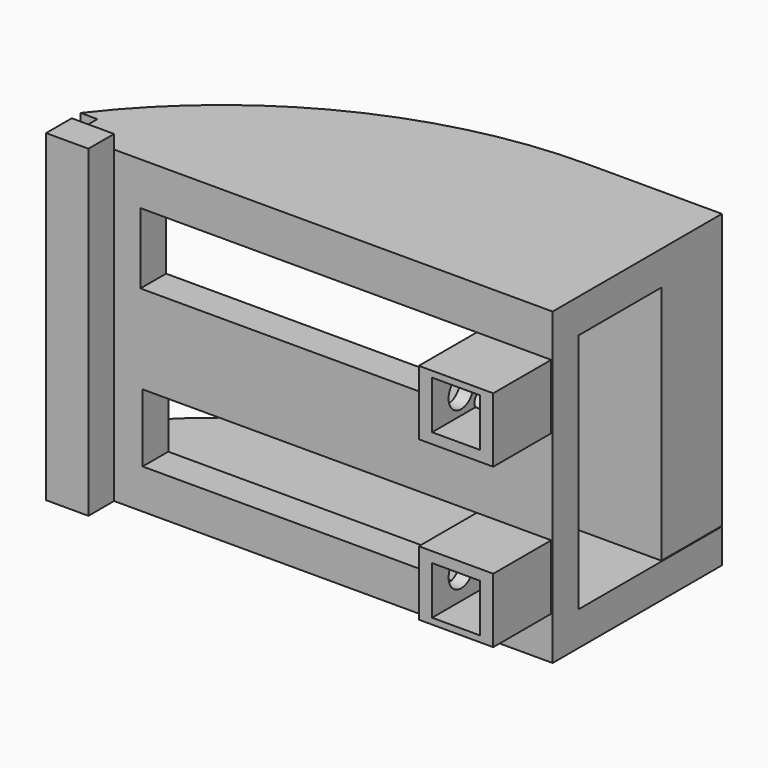
from build123d import *

# Parameters (mm, degrees)
F0_W         = 58.9547399431
F0_H         = 51.2344771996
F0_W_2       = 38.1
F0_H_2       = 38.1
F1_DEPTH     = 57.404
F2_R         = 12.4366404678
F3_DEPTH     = 25.4
F4_W         = 104.0811147541
F4_H         = 122.5580200553
F5_DEPTH     = 25.4
F6_DEPTH     = 25.4
F7_R         = 6.690453714
F8_DEPTH     = 25.4
F9_W         = 129.4811147541
F9_H         = 27.0336512476
F9_W_2       = 264.7406511664
F10_DEPTH    = 142.24
F11_T1_DEPTH = 1466.3511823856
F12_DEPTH    = 251.46
F16_W        = 33.5519401288
F16_H        = 256.0288235545
F17_DEPTH    = 25.4
F19_DEPTH    = 25.4
F20_W        = 66.9628661126
F20_H        = 59.9260473394
F21_DEPTH    = 190.5


# Not quite as in the source:
# - a fillet or chamfer that OpenCascade refuses, or shapes differently, is made with other operations: its cross-section is extruded or revolved along the edge and cut away or added
# - a feature of the source that left no trace in its solid (it failed there, or was rolled back) is left out


with BuildPart() as f1:
    # F0 (on Front) → F1 (new body)
    with BuildSketch(Plane.XZ):
        with Locations((-1.0527623817, -16.6687513702)):
            Rectangle(F0_W, F0_H)
        with Locations((-0.9248415082, -14.9141447619)):
            Rectangle(F0_W_2, F0_H_2, mode=Mode.SUBTRACT)
    extrude(amount=F1_DEPTH)

    # F2 (on face) → F3 (cut)
    with BuildSketch(Plane(origin=(-30.5301323533, 0, 0), x_dir=(0, -1, 0), z_dir=(-1, 0, 0))):
        with Locations((28.702, -17.1130020171)):
            Circle(F2_R)
    extrude(amount=-F3_DEPTH, mode=Mode.SUBTRACT)

    # F4 (on face) → F5 (join)
    with BuildSketch(Plane(origin=(0, 0, 0), x_dir=(-1, 0, 0), z_dir=(0, 1, 0))):
        with Locations((22.4943133071, -18.3081142604)):
            Rectangle(F4_W, F4_H)
    extrude(amount=F5_DEPTH)

    # F6 (add): a face of the model
    f6_faces = [f1.faces().sort_by_distance(p)[0] for p in [
        (-74.5348706841, 12.7, -18.3081142604),
    ]]
    extrude(f6_faces, amount=F6_DEPTH)

    # F7 (on face) → F8 (cut)
    with BuildSketch(Plane(origin=(-30.5301323533, 0, 0), x_dir=(0, -1, 0), z_dir=(-1, 0, 0))):
        with Locations((8.7604233995, -30.5925961584)):
            Circle(F7_R)
    extrude(amount=-F8_DEPTH, mode=Mode.SUBTRACT)

    # F9 (on face) → F10 (join)
    with BuildSketch(Plane(origin=(0, 25.4, 0), x_dir=(-1, 0, 0), z_dir=(0, 1, 0))):
        with Locations((35.1943133071, 29.4540701434)):
            Rectangle(F9_W, F9_H)
        with Locations((232.3051962674, 29.4540701434)):
            Rectangle(F9_W_2, F9_H)
    extrude(amount=F10_DEPTH)

    # F11: fillet of radius 362.4072547021 on 1 edges, made by hand

    # F11_s2 → F11_t1 (cut)
    with BuildSketch(Plane.XY.offset(-703.7215210494)):
        with BuildLine():
            ThreePointArc((-76.812015623, 167.64), (-237.3561028838, 130.139830949), (-364.6755218506, 25.4))
            Line((-364.6755218506, 25.4), (-364.6755218506, 167.64))
            Line((-364.6755218506, 167.64), (-76.812015623, 167.64))
        make_face()
    extrude(amount=F11_T1_DEPTH, mode=Mode.SUBTRACT)

    # F12 (add): a face of the model
    f12_faces = [f1.faces().sort_by_distance(p)[0] for p in [
        (-99.9348706841, 12.7, -18.3081142604),
    ]]
    extrude(f12_faces, amount=F12_DEPTH)

    # F15: F1 across face


with BuildPart() as f1_1:
    add(f1.part)
    add(f1.part.mirror(Plane(origin=(-160.9243133071, 12.7, -79.5871242881), x_dir=(1, 0, 0), z_dir=(0, 0, -1))))

    # F16 (on face) → F17 (join)
    with BuildSketch(Plane.XZ):
        with Locations((-334.6189006197, -74.1307325661)):
            Rectangle(F16_W, F16_H)
    extrude(amount=F17_DEPTH)

    # F18 (on face) → F19 (cut)
    with BuildSketch(Plane.XZ):
        Polygon((-295.2485382557, -116.8882586062), (-295.2485382557, -170.68554461), (-30.5301323533, -170.68554461), (-30.5301323533, -168.1227358058), (-30.5301323533, -116.8882586062), align=None)
        Polygon((-296.9728708267, 8.9484872296), (-296.9728708267, -47.0983237028), (-18.4958036989, -47.0983237028), (-18.4958036989, -42.28598997), (-30.5301323533, -42.28598997), (-30.5301323533, 8.9484872296), align=None)
    extrude(amount=-F19_DEPTH, mode=Mode.SUBTRACT)

    # F20 (on face) → F21 (join)
    with BuildSketch(Plane(origin=(0, 0, 15.9372445196), x_dir=(1, 0, 0), z_dir=(0, 0, -1))):
        with Locations((-3.9351889864, -137.6769763303)):
            Rectangle(F20_W, F20_H)
    extrude(amount=F21_DEPTH)


solid = f1_1.part
